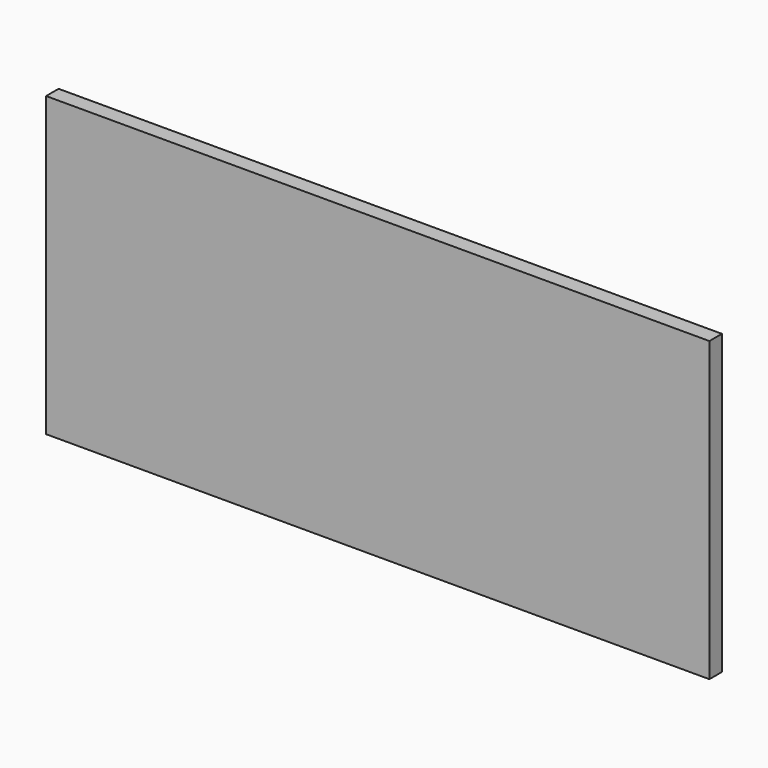
from build123d import *

# Parameters (mm, degrees)
F0_W     = 88.9
F0_H     = 63.5
F0_W_2   = 66.04
F0_H_2   = 12.192
F1_DEPTH = 6.35
F3_R     = 60.325
F3_R_2   = 7.9375
F4_DEPTH = 2.54
F6_W     = 127
F6_H     = 57
F7_DEPTH = 3


with BuildPart() as f1:
    # F0 (on Front) → F1 (new body)
    with BuildSketch(Plane.XZ):
        with Locations((10.876595974, 16.1719831105)):
            Rectangle(F0_W, F0_H)
        with Locations((11.8627893072, -0.3107596104)):
            Rectangle(F0_W_2, F0_H_2, mode=Mode.SUBTRACT)
        with Locations((10.9688239437, 30.9780669949)):
            Rectangle(F0_W_2, F0_H_2, mode=Mode.SUBTRACT)
    extrude(amount=F1_DEPTH)


with BuildPart() as f4:
    # F3 (on Front) → F4 (new body)
    with BuildSketch(Plane.XZ):
        with Locations((-8.6416769773, 16.2403918803)):
            Circle(F3_R)
        with Locations((-8.6416769773, 16.2403918803)):
            Circle(F3_R_2, mode=Mode.SUBTRACT)
    extrude(amount=F4_DEPTH)


with BuildPart() as f7:
    # F6 (on Front) → F7 (new body)
    with BuildSketch(Plane.XZ):
        with Locations((-11.0735092312, 8.7383504411)):
            Rectangle(F6_W, F6_H)
    extrude(amount=F7_DEPTH)


solid = f7.part
